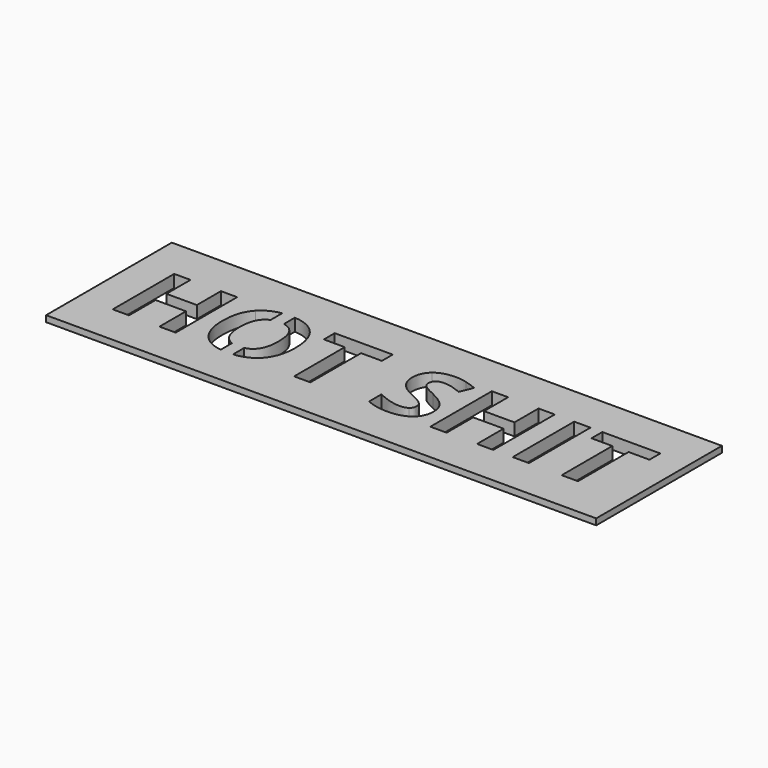
from build123d import *

# Parameters (mm, degrees)
F0_W     = 169
F0_H     = 44.45
F0_W_2   = 5.2673268342
F0_H_2   = 24.8363429365
F1_DEPTH = 4
F0_W_3   = 177.8
F0_H_3   = 50.8
F2_DEPTH = 2


with BuildPart() as f1:
    # F0 (on Top) → F1 (new body)
    with BuildSketch(Plane.XY):
        with Locations((2.6164503098, -12.6290581763)):
            Rectangle(F0_W, F0_H)
        Polygon((-55.1434959277, -0.2119976744), (-55.1434959277, -25.0483406109), (-60.3945152484, -25.0483406109), (-60.3945152484, -14.3288684571), (-70.2279458398, -14.3288684571), (-70.2279458398, -25.0483406109), (-75.495272674, -25.0483406109), (-75.495272674, -0.2119976744), (-70.2279458398, -0.2119976744), (-70.2279458398, -9.9475831853), (-60.3945152484, -9.9475831853), (-60.3945152484, -0.2119976744), align=None, mode=Mode.SUBTRACT)
        with BuildLine():
            Line((-40.7634110153, -0.0159870709), (-40.7634110153, 0))
            Line((-40.7634110153, 0), (-40.7634110153, 1.3887999812))
            Line((-40.7634110153, 1.3887999812), (-36.8744060397, 1.3887999812))
            Line((-36.8744060397, 1.3887999812), (-36.7738648248, 0.1308009128))
            add(Edge.make_bspline(
                [(-36.7738648248, 0.1308009128), (-32.0317465053, -0.2208247915), (-29.3667530507, -3.1174529818)],
                knots=[0.1213913838, 0.1213913838, 0.1213913838, 1, 1, 1], degree=2))
            add(Edge.make_bspline(
                [(-29.3667530507, -3.1174529818), (-26.3335555549, -6.4142886113), (-26.3335555549, -12.5948361969)],
                knots=[0, 0, 0, 1, 1, 1], degree=2))
            add(Edge.make_bspline(
                [(-26.3335555549, -12.5948361969), (-26.3335555549, -18.764512107), (-29.3912143208, -22.0776552498)],
                knots=[0, 0, 0, 1, 1, 1], degree=2))
            add(Edge.make_bspline(
                [(-29.3912143208, -22.0776552498), (-31.96172627, -24.8629477529), (-36.405085353, -25.3067011213)],
                knots=[0, 0, 0, 0.8406797965, 0.8406797965, 0.8406797965], degree=2))
            Line((-36.405085353, -25.3067011213), (-36.4003777504, -25.9454939514))
            Line((-36.4003777504, -25.9454939514), (-40.4519320428, -25.9454939514))
            Line((-40.4519320428, -25.9454939514), (-40.4519320428, -25.2426429066))
            add(Edge.make_bspline(
                [(-40.4519320428, -25.2426429066), (-44.5107206961, -24.6901841388), (-46.9217912458, -22.0776552498)],
                knots=[0.2114651326, 0.2114651326, 0.2114651326, 1, 1, 1], degree=2))
            add(Edge.make_bspline(
                [(-46.9217912458, -22.0776552498), (-49.9794500118, -18.764512107), (-49.9794500118, -12.5622211701)],
                knots=[0, 0, 0, 1, 1, 1], degree=2))
            add(Edge.make_bspline(
                [(-49.9794500118, -12.5622211701), (-49.9794500118, -6.3599302332), (-46.9136374891, -3.0902737928)],
                knots=[0, 0, 0, 1, 1, 1], degree=2))
            add(Edge.make_bspline(
                [(-46.9136374891, -3.0902737928), (-44.5972413071, -0.6198619073), (-40.7634110153, -0.0159870709)],
                knots=[0, 0, 0, 0.7555570228, 0.7555570228, 0.7555570228], degree=2))
        make_face(mode=Mode.SUBTRACT)
        Polygon((-11.6024351001, -4.5932829462), (-11.6024351001, -25.0483406109), (-16.8697619343, -25.0483406109), (-16.8697619343, -4.5932829462), (-23.6156366518, -4.5932829462), (-23.6156366518, -0.2119976744), (-4.8619962204, -0.2119976744), (-4.8619962204, -4.5932829462), align=None, mode=Mode.SUBTRACT)
        with BuildLine():
            add(Edge.make_bspline(
                [(21.3686391133, -14.0489228101), (22.6596505923, -15.7204429355), (22.6596505923, -18.1502624349)],
                knots=[0, 0, 0, 1, 1, 1], degree=2))
            add(Edge.make_bspline(
                [(22.6596505923, -18.1502624349), (22.6596505923, -21.5150460369), (20.2379848496, -23.4529222148)],
                knots=[0, 0, 0, 1, 1, 1], degree=2))
            add(Edge.make_bspline(
                [(20.2379848496, -23.4529222148), (17.816319107, -25.3907983927), (13.5056997267, -25.3907983927)],
                knots=[0, 0, 0, 1, 1, 1], degree=2))
            add(Edge.make_bspline(
                [(13.5056997267, -25.3907983927), (9.5266664525, -25.3907983927), (6.4717256055, -23.8905071582)],
                knots=[0, 0, 0, 1, 1, 1], degree=2))
            Line((6.4717256055, -23.8905071582), (6.4717256055, -18.9982531326))
            add(Edge.make_bspline(
                [(6.4717256055, -18.9982531326), (8.9830826719, -20.1234715585), (10.7252686888, -20.5800819342)],
                knots=[0, 0, 0, 1, 1, 1], degree=2))
            add(Edge.make_bspline(
                [(10.7252686888, -20.5800819342), (12.4674547057, -21.0366923099), (13.9133875621, -21.0366923099)],
                knots=[0, 0, 0, 1, 1, 1], degree=2))
            add(Edge.make_bspline(
                [(13.9133875621, -21.0366923099), (15.6419839845, -21.0366923099), (16.5687943305, -20.3762380165)],
                knots=[0, 0, 0, 1, 1, 1], degree=2))
            add(Edge.make_bspline(
                [(16.5687943305, -20.3762380165), (17.4956046764, -19.715783723), (17.4956046764, -18.4057468117)],
                knots=[0, 0, 0, 1, 1, 1], degree=2))
            add(Edge.make_bspline(
                [(17.4956046764, -18.4057468117), (17.4956046764, -17.6773445457), (17.0879168409, -17.1065815761)],
                knots=[0, 0, 0, 1, 1, 1], degree=2))
            add(Edge.make_bspline(
                [(17.0879168409, -17.1065815761), (16.6802290055, -16.5358186064), (15.8893146047, -16.0112602581)],
                knots=[0, 0, 0, 1, 1, 1], degree=2))
            add(Edge.make_bspline(
                [(15.8893146047, -16.0112602581), (15.0984002039, -15.4867019098), (12.6685807045, -14.3288684571)],
                knots=[0, 0, 0, 1, 1, 1], degree=2))
            add(Edge.make_bspline(
                [(12.6685807045, -14.3288684571), (10.3964005015, -13.2580084093), (9.2575924811, -12.2741217664)],
                knots=[0, 0, 0, 1, 1, 1], degree=2))
            add(Edge.make_bspline(
                [(9.2575924811, -12.2741217664), (8.1187844607, -11.2902351234), (7.439304735, -9.9801982122)],
                knots=[0, 0, 0, 1, 1, 1], degree=2))
            add(Edge.make_bspline(
                [(7.439304735, -9.9801982122), (6.7598250092, -8.6701613009), (6.7598250092, -6.9252573651)],
                knots=[0, 0, 0, 1, 1, 1], degree=2))
            add(Edge.make_bspline(
                [(6.7598250092, -6.9252573651), (6.7598250092, -3.6257038167), (8.9939543475, -1.7421860169)],
                knots=[0, 0, 0, 1, 1, 1], degree=2))
            add(Edge.make_bspline(
                [(8.9939543475, -1.7421860169), (11.2280836859, 0.141331783), (15.1690660954, 0.141331783)],
                knots=[0, 0, 0, 1, 1, 1], degree=2))
            add(Edge.make_bspline(
                [(15.1690660954, 0.141331783), (17.1042243544, 0.141331783), (18.8627178847, -0.3152785928)],
                knots=[0, 0, 0, 1, 1, 1], degree=2))
            add(Edge.make_bspline(
                [(18.8627178847, -0.3152785928), (20.621211415, -0.7718889685), (22.5400621606, -1.6035721528)],
                knots=[0, 0, 0, 1, 1, 1], degree=2))
            Line((22.5400621606, -1.6035721528), (20.844080765, -5.7021938587))
            add(Edge.make_bspline(
                [(20.844080765, -5.7021938587), (18.854564128, -4.8868181878), (17.5553988923, -4.5633858383)],
                knots=[0, 0, 0, 1, 1, 1], degree=2))
            add(Edge.make_bspline(
                [(17.5553988923, -4.5633858383), (16.2562336566, -4.2399534888), (15.0005551234, -4.2399534888)],
                knots=[0, 0, 0, 1, 1, 1], degree=2))
            add(Edge.make_bspline(
                [(15.0005551234, -4.2399534888), (13.5056997267, -4.2399534888), (12.7066315692, -4.935740728)],
                knots=[0, 0, 0, 1, 1, 1], degree=2))
            add(Edge.make_bspline(
                [(12.7066315692, -4.935740728), (11.9075634117, -5.6315279672), (11.9075634117, -6.7513105553)],
                knots=[0, 0, 0, 1, 1, 1], degree=2))
            add(Edge.make_bspline(
                [(11.9075634117, -6.7513105553), (11.9075634117, -7.4470977945), (12.2309957611, -7.966220305)],
                knots=[0, 0, 0, 1, 1, 1], degree=2))
            add(Edge.make_bspline(
                [(12.2309957611, -7.966220305), (12.5544281106, -8.4853428155), (13.2583691065, -8.9691323802)],
                knots=[0, 0, 0, 1, 1, 1], degree=2))
            add(Edge.make_bspline(
                [(13.2583691065, -8.9691323802), (13.9623101024, -9.452921945), (16.5932556006, -10.7086004782)],
                knots=[0, 0, 0, 1, 1, 1], degree=2))
            add(Edge.make_bspline(
                [(16.5932556006, -10.7086004782), (20.0776276343, -12.3774026847), (21.3686391133, -14.0489228101)],
                knots=[0, 0, 0, 1, 1, 1], degree=2))
        make_face(mode=Mode.SUBTRACT)
        Polygon((47.5123010422, -0.2119976744), (47.5123010422, -25.0483406109), (42.2612817214, -25.0483406109), (42.2612817214, -14.3288684571), (32.42785113, -14.3288684571), (32.42785113, -25.0483406109), (27.1605242958, -25.0483406109), (27.1605242958, -0.2119976744), (32.42785113, -0.2119976744), (32.42785113, -9.9475831853), (42.2612817214, -9.9475831853), (42.2612817214, -0.2119976744), align=None, mode=Mode.SUBTRACT)
        with Locations((56.4134854498, -12.6301691427)):
            Rectangle(F0_W_2, F0_H_2, mode=Mode.SUBTRACT)
        Polygon((74.8817443963, -4.5932829462), (74.8817443963, -25.0483406109), (69.6144175621, -25.0483406109), (69.6144175621, -4.5932829462), (62.8685428446, -4.5932829462), (62.8685428446, -0.2119976744), (81.622183276, -0.2119976744), (81.622183276, -4.5932829462), align=None, mode=Mode.SUBTRACT)
        with BuildLine():
            Line((-40.7634110153, 1.3887999812), (-40.7634110153, 0))
            Line((-40.7634110153, 0), (-40.7634110153, -0.0159870709))
            add(Edge.make_bspline(
                [(-40.7634110153, -0.0159870709), (-39.5230640096, 0.1793826476), (-38.1238877565, 0.1793826476)],
                knots=[0.7555570228, 0.7555570228, 0.7555570228, 1, 1, 1], degree=2))
            add(Edge.make_bspline(
                [(-38.1238877565, 0.1793826476), (-37.429051098, 0.1793826476), (-36.7738648248, 0.1308009128)],
                knots=[0, 0, 0, 0.1213913838, 0.1213913838, 0.1213913838], degree=2))
            Line((-36.7738648248, 0.1308009128), (-36.8744060397, 1.3887999812))
            Line((-36.8744060397, 1.3887999812), (-40.7634110153, 1.3887999812))
        make_face()
        with BuildLine():
            add(Edge.make_bspline(
                [(-40.7634110153, -0.0159870709), (-39.5230640096, 0.1793826476), (-38.1238877565, 0.1793826476)],
                knots=[0.7555570228, 0.7555570228, 0.7555570228, 1, 1, 1], degree=2))
            Line((-40.7634110153, -0.0159870709), (-40.7634110153, -4.6859490545))
            add(Edge.make_bspline(
                [(-38.1238877565, -4.207338462), (-39.6186682979, -4.207338462), (-40.7634110153, -4.6859490545)],
                knots=[0, 0, 0, 0.475754722, 0.475754722, 0.475754722], degree=2))
            add(Edge.make_bspline(
                [(-36.7634110153, -4.3185824581), (-37.4020860912, -4.207338462), (-38.1238877565, -4.207338462)],
                knots=[0.8848345835, 0.8848345835, 0.8848345835, 1, 1, 1], degree=2))
            Line((-36.7634110153, -4.3185824581), (-36.7634110153, 0))
            Line((-36.7634110153, 0), (-36.7738648248, 0.1308009128))
            add(Edge.make_bspline(
                [(-38.1238877565, 0.1793826476), (-37.429051098, 0.1793826476), (-36.7738648248, 0.1308009128)],
                knots=[0, 0, 0, 0.1213913838, 0.1213913838, 0.1213913838], degree=2))
        make_face()
        with BuildLine():
            add(Edge.make_bspline(
                [(-38.1238877565, -4.207338462), (-39.6186682979, -4.207338462), (-40.7634110153, -4.6859490545)],
                knots=[0, 0, 0, 0.475754722, 0.475754722, 0.475754722], degree=2))
            Line((-40.7634110153, -4.6859490545), (-40.7634110153, -4.7359894961))
            Line((-40.7634110153, -4.7359894961), (-36.7634110153, -4.9380864948))
            Line((-36.7634110153, -4.9380864948), (-36.7634110153, -4.3185824581))
            add(Edge.make_bspline(
                [(-36.7634110153, -4.3185824581), (-37.4020860912, -4.207338462), (-38.1238877565, -4.207338462)],
                knots=[0.8848345835, 0.8848345835, 0.8848345835, 1, 1, 1], degree=2))
        make_face()
        with BuildLine():
            Line((-40.7634110153, -4.7359894961), (-40.7634110153, -4.6859490545))
            add(Edge.make_bspline(
                [(-40.7634110153, -4.6859490545), (-42.0248298439, -5.2133412831), (-42.8612204046, -6.3218793686)],
                knots=[0.475754722, 0.475754722, 0.475754722, 1, 1, 1], degree=2))
            add(Edge.make_bspline(
                [(-42.8612204046, -6.3218793686), (-44.4566388007, -8.4364202752), (-44.4566388007, -12.5948361969)],
                knots=[0, 0, 0, 1, 1, 1], degree=2))
            add(Edge.make_bspline(
                [(-44.4566388007, -12.5948361969), (-44.4566388007, -16.7586879565), (-42.877527918, -18.8650751064)],
                knots=[0, 0, 0, 1, 1, 1], degree=2))
            add(Edge.make_bspline(
                [(-42.877527918, -18.8650751064), (-41.9401032757, -20.115512452), (-40.4519320428, -20.6236391757)],
                knots=[0, 0, 0, 0.5936407966, 0.5936407966, 0.5936407966], degree=2))
            Line((-40.4519320428, -20.6236391757), (-40.4519320428, -18.9498923719))
            Line((-40.4519320428, -18.9498923719), (-36.4519320428, -18.9498923719))
            Line((-36.4519320428, -18.9498923719), (-36.4383714184, -20.7899860206))
            add(Edge.make_bspline(
                [(-36.4383714184, -20.7899860206), (-31.856366766, -19.7385151508), (-31.856366766, -12.5948361969)],
                knots=[0.1471889872, 0.1471889872, 0.1471889872, 1, 1, 1], degree=2))
            add(Edge.make_bspline(
                [(-31.856366766, -12.5948361969), (-31.856366766, -5.173288132), (-36.7634110153, -4.3185824581)],
                knots=[0, 0, 0, 0.8848345835, 0.8848345835, 0.8848345835], degree=2))
            Line((-36.7634110153, -4.3185824581), (-36.7634110153, -4.9380864948))
            Line((-36.7634110153, -4.9380864948), (-40.7634110153, -4.7359894961))
        make_face()
        with BuildLine():
            add(Edge.make_bspline(
                [(-38.1565027833, -25.3907983927), (-39.3634674537, -25.3907983927), (-40.4519320428, -25.2426429066)],
                knots=[0, 0, 0, 0.2114651326, 0.2114651326, 0.2114651326], degree=2))
            Line((-40.4519320428, -25.2426429066), (-40.4519320428, -25.9454939514))
            Line((-40.4519320428, -25.9454939514), (-36.4003777504, -25.9454939514))
            Line((-36.4003777504, -25.9454939514), (-36.405085353, -25.3067011213))
            add(Edge.make_bspline(
                [(-36.405085353, -25.3067011213), (-37.2471620585, -25.3907983927), (-38.1565027833, -25.3907983927)],
                knots=[0.8406797965, 0.8406797965, 0.8406797965, 1, 1, 1], degree=2))
        make_face()
        with BuildLine():
            Line((-40.4519320428, -25.0483406109), (-40.4519320428, -25.2426429066))
            add(Edge.make_bspline(
                [(-38.1565027833, -25.3907983927), (-39.3634674537, -25.3907983927), (-40.4519320428, -25.2426429066)],
                knots=[0, 0, 0, 0.2114651326, 0.2114651326, 0.2114651326], degree=2))
            add(Edge.make_bspline(
                [(-36.405085353, -25.3067011213), (-37.2471620585, -25.3907983927), (-38.1565027833, -25.3907983927)],
                knots=[0.8406797965, 0.8406797965, 0.8406797965, 1, 1, 1], degree=2))
            Line((-36.405085353, -25.3067011213), (-36.4383714184, -20.7899860206))
            add(Edge.make_bspline(
                [(-38.1565027833, -20.9714622563), (-37.2291921439, -20.9714622563), (-36.4383714184, -20.7899860206)],
                knots=[0, 0, 0, 0.1471889872, 0.1471889872, 0.1471889872], degree=2))
            add(Edge.make_bspline(
                [(-40.4519320428, -20.6236391757), (-39.4332485559, -20.9714622563), (-38.1565027833, -20.9714622563)],
                knots=[0.5936407966, 0.5936407966, 0.5936407966, 1, 1, 1], degree=2))
            Line((-40.4519320428, -20.6236391757), (-40.4519320428, -25.0483406109))
        make_face()
        with BuildLine():
            add(Edge.make_bspline(
                [(-38.1565027833, -20.9714622563), (-37.2291921439, -20.9714622563), (-36.4383714184, -20.7899860206)],
                knots=[0, 0, 0, 0.1471889872, 0.1471889872, 0.1471889872], degree=2))
            Line((-36.4383714184, -20.7899860206), (-36.4519320428, -18.9498923719))
            Line((-36.4519320428, -18.9498923719), (-40.4519320428, -18.9498923719))
            Line((-40.4519320428, -18.9498923719), (-40.4519320428, -20.6236391757))
            add(Edge.make_bspline(
                [(-40.4519320428, -20.6236391757), (-39.4332485559, -20.9714622563), (-38.1565027833, -20.9714622563)],
                knots=[0.5936407966, 0.5936407966, 0.5936407966, 1, 1, 1], degree=2))
        make_face()
    extrude(amount=-F1_DEPTH)

    # F0 (on Top) → F2 (join)
    with BuildSketch(Plane.XY):
        with Locations((2.2549219429, -12.638609002)):
            Rectangle(F0_W_3, F0_H_3)
        with Locations((2.6164503098, -12.6290581763)):
            Rectangle(F0_W, F0_H, mode=Mode.SUBTRACT)
    extrude(amount=-F2_DEPTH)


solid = f1.part
